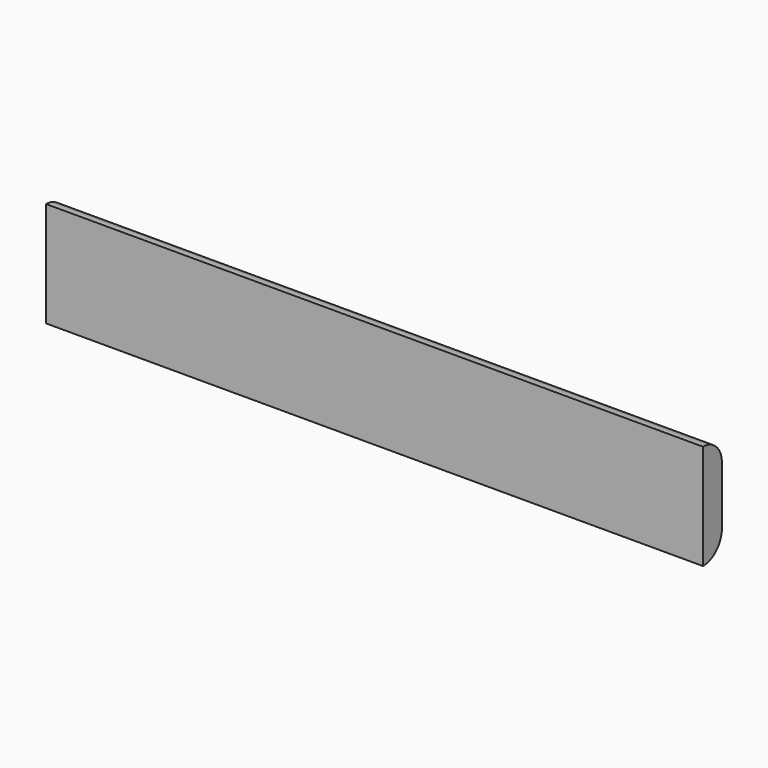
from build123d import *

# Parameters (mm, degrees)
F0_W     = 500
F0_H     = 80
F1_DEPTH = 18
F2_R     = 17.99999


# Not quite as in the source:
# - a fillet or chamfer is up to 0.001 mm smaller than in the source, because OpenCascade refuses the exact size


with BuildPart() as f1:
    # F0 (on Front) → F1 (new body)
    with BuildSketch(Plane.XZ):
        with Locations((48.9213317633, -38.1839564443)):
            Rectangle(F0_W, F0_H)
    extrude(amount=F1_DEPTH)

    # F2 (radius 18 in the source; OpenCascade refuses exactly that, so slightly less here)
    f2_edges = [f1.edges().sort_by_distance(p)[0] for p in [
        (48.921332, 0, -78.183956),
        (48.921332, 0, 1.816044),
    ]]
    fillet(f2_edges, radius=F2_R)


solid = f1.part
